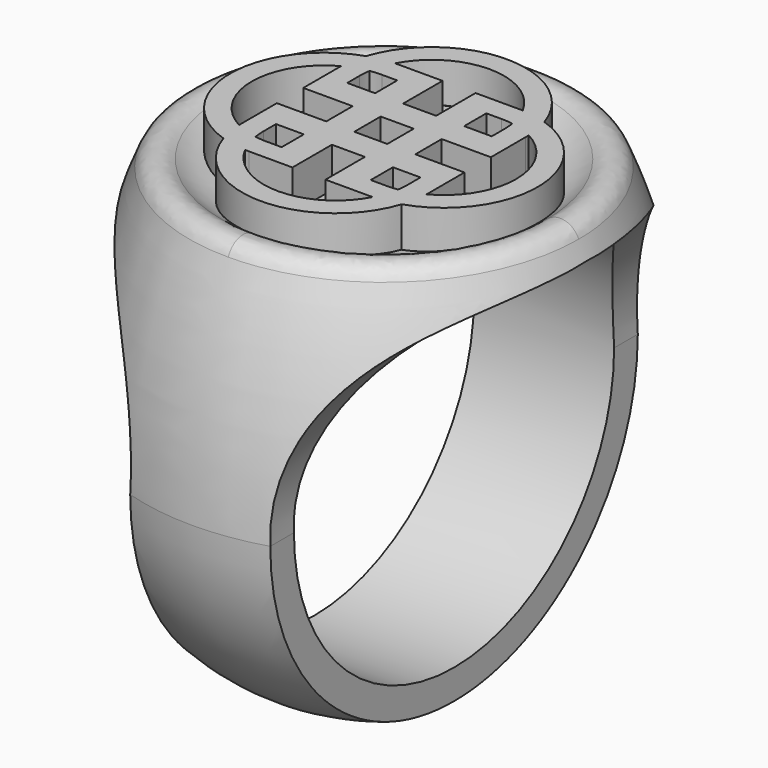
from build123d import *

# Parameters (mm, degrees)
F2_R         = 10
F3_DEPTH     = 12.5
F5_DEPTH     = 12.5
F6_R         = 9
F6_W         = 1.65
F6_H         = 1.65
F7_DEPTH     = 2
F8_T4_ANGLE  = 269.9999991059
F8_S5_R      = 3.61
F8_T6_DEPTH  = 16
F8_S7_R      = 3.61
F8_T8_DEPTH  = 16
F8_S9_R      = 3.61
F8_T10_DEPTH = 16
F8_S11_R     = 3.61
F8_T12_DEPTH = 16
F8_T16_ANGLE = 90.0000008941
F8_S17_R     = 3.61
F8_T18_DEPTH = 9
F8_S19_R     = 3.61
F8_T20_DEPTH = 9
F9_R         = 1


# Not quite as in the source:
# - a fillet or chamfer that OpenCascade refuses, or shapes differently, is made with other operations: its cross-section is extruded or revolved along the edge and cut away or added


with BuildPart() as f1:
    # F0 (on Right) → F1 (revolve)
    with BuildSketch(Plane.YZ):
        with BuildLine():
            Line((0, -24.5), (0, 0))
            Line((0, 0), (-9, 0))
            ThreePointArc((-9, 0), (-11.177394056, -6.0874254266), (-12, -12.5))
            ThreePointArc((-12, -12.5), (-8.4852813742, -20.9852813742), (0, -24.5))
        make_face()
    revolve(axis=Axis((0, 0, -12.25), (0, 0, -1)))

    # F2 (on Right) → F3 (cut, symmetric)
    with BuildSketch(Plane.YZ):
        with Locations((0, -12.5)):
            Circle(F2_R)
    extrude(amount=F3_DEPTH, both=True, mode=Mode.SUBTRACT)

    # F4 (on Front) → F5 (cut, symmetric)
    with BuildSketch(Plane.XZ):
        with BuildLine():
            Line((3.5, -12.5), (3.5, -26.5))
            Line((3.5, -26.5), (11.6508146748, -26.5))
            Line((11.6508146748, -26.5), (11.6508146748, -2.5))
            Line((11.6508146748, -2.5), (10.1532964036, -2.5))
            ThreePointArc((10.1532964036, -2.5), (5.1580549578, -6.3898354571), (3.5, -12.5))
        make_face()
        with BuildLine():
            Line((-11.6508146748, -26.5), (-3.5, -26.5))
            Line((-3.5, -26.5), (-3.5, -12.5))
            ThreePointArc((-3.5, -12.5), (-5.1580549578, -6.3898354571), (-10.1532964036, -2.5))
            Line((-10.1532964036, -2.5), (-11.6508146748, -2.5))
            Line((-11.6508146748, -2.5), (-11.6508146748, -26.5))
        make_face()
    extrude(amount=F5_DEPTH, both=True, mode=Mode.SUBTRACT)

    # F6 (on face) → F7 (cut)
    with BuildSketch(Plane.XY):
        Circle(F6_R)
        with BuildLine():
            ThreePointArc((-4.4621427539, -4.4514560696), (-7.682, 0), (-4.4621427539, 4.4514560696))
            ThreePointArc((-4.4621427539, 4.4514560696), (-0.0099507904, 7.6819991802), (4.4460594172, 4.4567247579))
            ThreePointArc((4.4460594172, 4.4567247579), (7.682, 0), (4.4460594172, -4.4567247579))
            ThreePointArc((4.4460594172, -4.4567247579), (-0.0099507904, -7.6819991802), (-4.4621427539, -4.4514560696))
        make_face(mode=Mode.SUBTRACT)
        with BuildLine():
            ThreePointArc((4.6755534697, -3.1949710539), (6.605, 0), (4.6755534697, 3.1949710539))
            ThreePointArc((4.6755534697, 3.1949710539), (4.6787542206, 3.0950082956), (4.6798212996, 2.995))
            Line((4.6798212996, 2.995), (4.6798212996, 0.825))
            Line((4.6798212996, 0.825), (2.225, 0.825))
            Line((2.225, 0.825), (2.225, -0.825))
            Line((2.225, -0.825), (4.6798212996, -0.825))
            Line((4.6798212996, -0.825), (4.6798212996, -2.995))
            ThreePointArc((4.6798212996, -2.995), (4.6787542206, -3.0950082956), (4.6755534697, -3.1949710539))
        make_face()
        with BuildLine():
            ThreePointArc((-3.198442533, 4.6825826352), (-3.0967452424, 4.6858955287), (-2.995, 4.687))
            Line((-2.995, 4.687), (-0.825, 4.687))
            Line((-0.825, 4.687), (-0.825, 2.225))
            Line((-0.825, 2.225), (0.825, 2.225))
            Line((0.825, 2.225), (0.825, 4.687))
            Line((0.825, 4.687), (2.995, 4.687))
            ThreePointArc((2.995, 4.687), (3.0893991057, 4.6860492751), (3.183759915, 4.6831974862))
            ThreePointArc((3.183759915, 4.6831974862), (-0.0075264819, 6.6049999832), (-3.198442533, 4.6825826352))
        make_face()
        with BuildLine():
            ThreePointArc((-2.995, -4.687), (-3.0967452424, -4.6858955287), (-3.198442533, -4.6825826352))
            ThreePointArc((-3.198442533, -4.6825826352), (-0.0075264819, -6.6049999832), (3.183759915, -4.6831974862))
            ThreePointArc((3.183759915, -4.6831974862), (3.0893991057, -4.6860492751), (2.995, -4.687))
            Line((2.995, -4.687), (0.825, -4.687))
            Line((0.825, -4.687), (0.825, -2.225))
            Line((0.825, -2.225), (-0.825, -2.225))
            Line((-0.825, -2.225), (-0.825, -4.687))
            Line((-0.825, -4.687), (-2.995, -4.687))
        make_face()
        with BuildLine():
            ThreePointArc((-4.6941787004, 2.995), (-4.6931929385, 3.0911226351), (-4.6902360672, 3.1872048375))
            ThreePointArc((-4.6902360672, 3.1872048375), (-6.605, 0), (-4.6902360672, -3.1872048375))
            ThreePointArc((-4.6902360672, -3.1872048375), (-4.6931929385, -3.0911226351), (-4.6941787004, -2.995))
            Line((-4.6941787004, -2.995), (-4.6941787004, -0.825))
            Line((-4.6941787004, -0.825), (-2.225, -0.825))
            Line((-2.225, -0.825), (-2.225, 0.825))
            Line((-2.225, 0.825), (-4.6941787004, 0.825))
            Line((-4.6941787004, 0.825), (-4.6941787004, 2.995))
        make_face()
        Rectangle(F6_W, F6_H)
        with BuildLine():
            ThreePointArc((-2.995, 3.61), (-3.2844938841, 3.5983737009), (-3.5721230909, 3.5635696903))
            ThreePointArc((-3.5721230909, 3.5635696903), (-3.6058971702, 3.2801760424), (-3.6171787004, 2.995))
            Line((-3.6171787004, 2.995), (-3.6171787004, 2.225))
            Line((-3.6171787004, 2.225), (-2.225, 2.225))
            Line((-2.225, 2.225), (-2.225, 3.61))
            Line((-2.225, 3.61), (-2.995, 3.61))
        make_face()
        with BuildLine():
            ThreePointArc((-3.6171787004, -2.995), (-3.6058971702, -3.2801760424), (-3.5721230909, -3.5635696903))
            ThreePointArc((-3.5721230909, -3.5635696903), (-3.2844938841, -3.5983737009), (-2.995, -3.61))
            Line((-2.995, -3.61), (-2.225, -3.61))
            Line((-2.225, -3.61), (-2.225, -2.225))
            Line((-2.225, -2.225), (-3.6171787004, -2.225))
            Line((-3.6171787004, -2.225), (-3.6171787004, -2.995))
        make_face()
        with BuildLine():
            ThreePointArc((3.6028212996, 2.995), (3.5914453781, 3.2813647003), (3.5573893097, 3.5659246016))
            ThreePointArc((3.5573893097, 3.5659246016), (3.2770568987, 3.5989642824), (2.995, 3.61))
            Line((2.995, 3.61), (2.225, 3.61))
            Line((2.225, 3.61), (2.225, 2.225))
            Line((2.225, 2.225), (3.6028212996, 2.225))
            Line((3.6028212996, 2.225), (3.6028212996, 2.995))
        make_face()
        with BuildLine():
            ThreePointArc((2.995, -3.61), (3.2770568987, -3.5989642824), (3.5573893097, -3.5659246016))
            ThreePointArc((3.5573893097, -3.5659246016), (3.5914453781, -3.2813647003), (3.6028212996, -2.995))
            Line((3.6028212996, -2.995), (3.6028212996, -2.225))
            Line((3.6028212996, -2.225), (2.225, -2.225))
            Line((2.225, -2.225), (2.225, -3.61))
            Line((2.225, -3.61), (2.995, -3.61))
        make_face()
    extrude(amount=-F7_DEPTH, mode=Mode.SUBTRACT)

    # F8: fillet of radius 3 on 1 edges, made by hand


with BuildPart() as f8_tool2:
    # F8_s3 → F8_t4 (revolve)
    with BuildSketch(Plane.XZ):
        with BuildLine():
            ThreePointArc((9, 0), (7.9036236828, -1.4494897428), (6.1715728753, -2))
            Line((6.1715728753, -2), (9, -2))
            Line((9, -2), (9, 0))
        make_face()
    revolve(axis=Axis((0, 0, -2), (0, 0, 1)), revolution_arc=F8_T4_ANGLE)

    # F8_s5 → F8_t6 (cut, symmetric)
    with BuildSketch(Plane.XY.offset(-0.5)):
        with Locations((2.995, 0)):
            Circle(F8_S5_R)
    extrude(amount=F8_T6_DEPTH, both=True, mode=Mode.SUBTRACT)

    # F8_s7 → F8_t8 (cut, symmetric)
    with BuildSketch(Plane.XY.offset(-0.5)):
        with Locations((-0.0071787004, -2.995)):
            Circle(F8_S7_R)
    extrude(amount=F8_T8_DEPTH, both=True, mode=Mode.SUBTRACT)

    # F8_s9 → F8_t10 (cut, symmetric)
    with BuildSketch(Plane.XY.offset(-0.5)):
        with Locations((-2.995, 0)):
            Circle(F8_S9_R)
    extrude(amount=F8_T10_DEPTH, both=True, mode=Mode.SUBTRACT)

    # F8_s11 → F8_t12 (cut, symmetric)
    with BuildSketch(Plane.XY.offset(-0.5)):
        with Locations((-0.0071787004, 2.995)):
            Circle(F8_S11_R)
    extrude(amount=F8_T12_DEPTH, both=True, mode=Mode.SUBTRACT)


with BuildPart() as f1_1:
    add(f1.part)

    # F8_t1: union F8_tool2
    add(f8_tool2.part)


with BuildPart() as f8_tool14:
    # F8_s15 → F8_t16 (revolve)
    with BuildSketch(Plane.YZ):
        with BuildLine():
            ThreePointArc((-9, 0), (-7.9036236828, -1.4494897428), (-6.1715728753, -2))
            Line((-6.1715728753, -2), (-9, -2))
            Line((-9, -2), (-9, 0))
        make_face()
    revolve(axis=Axis((0, 0, -2), (0, 0, 1)), revolution_arc=F8_T16_ANGLE)

    # F8_s17 → F8_t18 (cut, symmetric)
    with BuildSketch(Plane.XY.offset(-0.5)):
        with Locations((2.995, 0)):
            Circle(F8_S17_R)
    extrude(amount=F8_T18_DEPTH, both=True, mode=Mode.SUBTRACT)

    # F8_s19 → F8_t20 (cut, symmetric)
    with BuildSketch(Plane.XY.offset(-0.5)):
        with Locations((-0.0071787004, -2.995)):
            Circle(F8_S19_R)
    extrude(amount=F8_T20_DEPTH, both=True, mode=Mode.SUBTRACT)


with BuildPart() as f1_2:
    add(f1_1.part)

    # F8_t13: union F8_tool14
    add(f8_tool14.part)

    # F9
    f9_edges = [f1_2.edges().sort_by_distance(p)[0] for p in [
        (-6.363961, 6.363961, 0),
        (6.363961, -6.363961, 0),
    ]]
    fillet(f9_edges, radius=F9_R)


solid = f1_2.part
